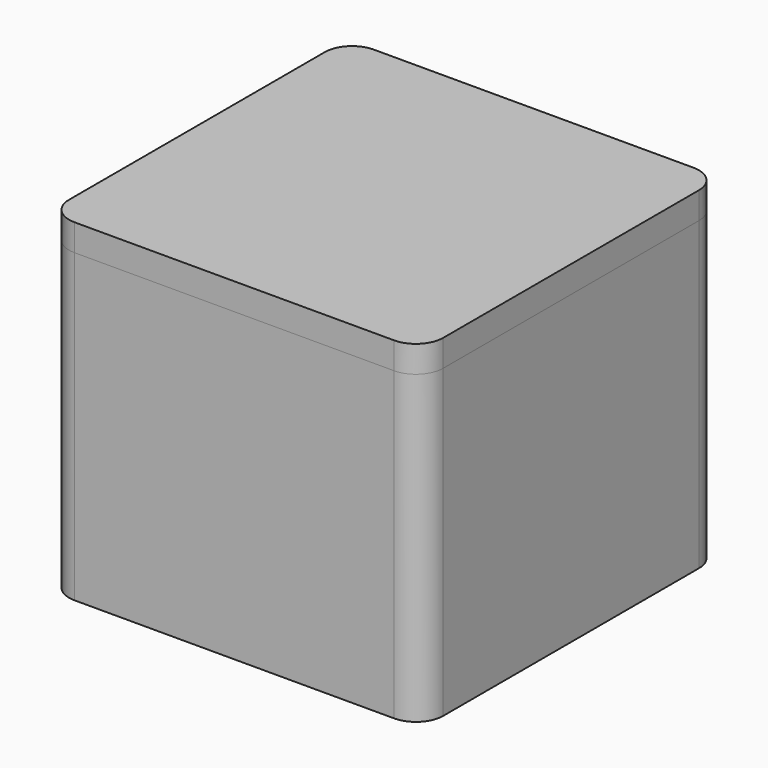
from build123d import *

# Parameters (mm, degrees)
F0_W      = 69.85
F0_H      = 69.85
F0_W_2    = 63.5
F0_H_2    = 63.5
F1_DEPTH  = 44.45
F0_W_3    = 44.45
F0_H_3    = 44.45
F2_W      = 69.85
F2_H      = 69.85
F3_DEPTH  = 5
F4_W      = 69.85
F4_H      = 69.85
F4_W_2    = 63.5
F4_H_2    = 63.5
F5_DEPTH  = 12.7
F6_R      = 5.08
F6_2_R    = 5.08
F7_R      = 2.54
F8_R      = 5.08
F9_R      = 3.175
F10_DEPTH = 12.7


with BuildPart() as f1:
    # F0 (on Top) → F1 (new body)
    with BuildSketch(Plane.XY):
        with Locations((22.225, 22.225)):
            Rectangle(F0_W, F0_H)
        with Locations((22.225, 22.225)):
            Rectangle(F0_W_2, F0_H_2, mode=Mode.SUBTRACT)
    extrude(amount=F1_DEPTH)

    # F4 (on face) → F5 (join)
    with BuildSketch(Plane(origin=(0, 0, 0), x_dir=(1, 0, 0), z_dir=(0, 0, -1))):
        with Locations((22.225, -22.225)):
            Rectangle(F4_W, F4_H)
        with Locations((22.225, -22.225)):
            Rectangle(F4_W_2, F4_H_2, mode=Mode.SUBTRACT)
    extrude(amount=F5_DEPTH)

    # F6
    f6_edges = [f1.edges().sort_by_distance(p)[0] for p in [
        (53.975, -9.525, 15.875),
        (-9.525, -9.525, 15.875),
        (-9.525, 53.975, 15.875),
        (53.975, 53.975, 15.875),
        (-12.7, -12.7, 15.875),
        (-12.7, 57.15, 15.875),
        (57.15, 57.15, 15.875),
        (57.15, -12.7, 15.875),
    ]]
    fillet(f6_edges, radius=F6_R)


with BuildPart() as f1b:
    # F0 (on Top) → F1, piece 2 (new body)
    with BuildSketch(Plane.XY):
        with Locations((22.225, 22.225)):
            Rectangle(F0_W_3, F0_H_3)
    extrude(amount=F1_DEPTH)

    # F2 (on face) → F3 (join)
    with BuildSketch(Plane.XY.offset(44.45)):
        with Locations((22.225, 22.225)):
            Rectangle(F2_W, F2_H)
    extrude(amount=F3_DEPTH)

    # F6#2
    f6_2_edges = [f1b.edges().sort_by_distance(p)[0] for p in [
        (-12.7, -12.7, 46.95),
    ]]
    fillet(f6_2_edges, radius=F6_2_R)

    # F7
    f7_edges = [f1b.edges().sort_by_distance(p)[0] for p in [
        (0, 0, 22.225),
        (44.45, 0, 22.225),
        (0, 44.45, 22.225),
        (44.45, 44.45, 22.225),
        (44.45, 22.225, 0),
        (22.225, 44.45, 0),
        (22.225, 0, 0),
        (0, 22.225, 0),
    ]]
    fillet(f7_edges, radius=F7_R)

    # F8
    f8_edges = [f1b.edges().sort_by_distance(p)[0] for p in [
        (57.15, 57.15, 46.95),
        (-12.7, 57.15, 46.95),
        (57.15, -12.7, 46.95),
    ]]
    fillet(f8_edges, radius=F8_R)

    # F9 (on face) → F10 (join)
    with BuildSketch(Plane(origin=(0, 0, 0), x_dir=(1, 0, 0), z_dir=(0, 0, -1))):
        with Locations((22.225, -22.225)):
            Circle(F9_R)
    extrude(amount=F10_DEPTH)


solid = Compound([f1.part, f1b.part])
